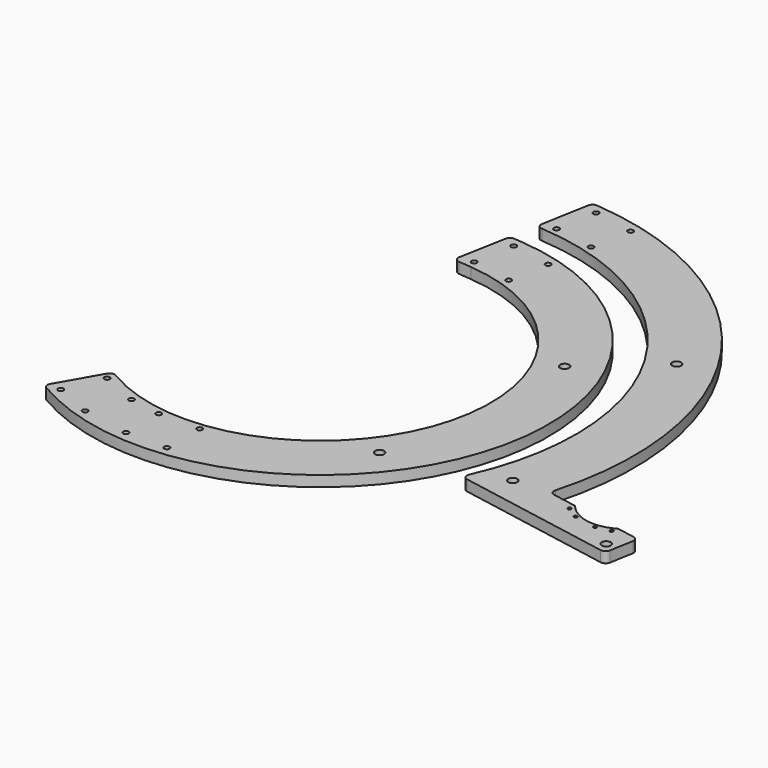
from build123d import *

# Parameters (mm, degrees)
F0_R     = 1.6
F0_R_2   = 2.65
F1_DEPTH = 6.3
F2_R     = 2.65
F2_R_2   = 1
F2_R_3   = 1.6
F3_DEPTH = 6.3


# Not quite as in the source:
# - a feature names something its author has since deleted; it is built from what else it names


with BuildPart() as f1:
    # F0 (on Top) → F1 (new body)
    with BuildSketch(Plane.XY):
        with BuildLine():
            ThreePointArc((8.7155742748, 99.6194698092), (95.3716950748, -30.0705799504), (-50, -86.6025403784))
            Line((-50, -86.6025403784), (-50.3901909826, -86.3515001966))
            Line((-50.3901909826, -86.3515001966), (-51.0879005816, -85.9026093909))
            ThreePointArc((-51.0879005816, -85.9026093909), (-53.4238831161, -85.5114532249), (-55.315580219, -86.9366899133))
            Line((-55.315580219, -86.9366899133), (-69.2410233648, -111.2966505134))
            ThreePointArc((-69.2410233648, -111.2966505134), (-69.5365488426, -113.5536105543), (-68.1625734678, -115.3683820561))
            ThreePointArc((-68.1625734678, -115.3683820561), (127.5940316963, -40.9360852487), (11.6788695282, 133.4900895443))
            Line((11.6788695282, 133.4900895443), (6.777103854, 133.918938472))
            ThreePointArc((6.777103854, 133.918938472), (4.6955895728, 133.3151874379), (3.563981512, 131.4667610231))
            Line((3.563981512, 131.4667610231), (-1.4639765495, 103.799694903))
            ThreePointArc((-1.4639765495, 103.799694903), (-0.8971544959, 101.4432412046), (1.226211336, 100.2747041633))
            Line((1.226211336, 100.2747041633), (8.7155742748, 99.6194698092))
        make_face()
        with Locations((-62.0446017151, -112.5987006942)):
            Circle(F0_R, mode=Mode.SUBTRACT)
        with Locations((-40.0351599298, -122.1686783484)):
            Circle(F0_R, mode=Mode.SUBTRACT)
        with Locations((-52.4746240608, -90.5892589089)):
            Circle(F0_R, mode=Mode.SUBTRACT)
        with Locations((-30.4651822756, -100.1592365632)):
            Circle(F0_R, mode=Mode.SUBTRACT)
        with Locations((-12, -127.3053725612)):
            Circle(F0_R, mode=Mode.SUBTRACT)
        with Locations((-12, -103.3053725612)):
            Circle(F0_R, mode=Mode.SUBTRACT)
        with Locations((12, -127.3053725612)):
            Circle(F0_R, mode=Mode.SUBTRACT)
        with Locations((12, -103.3053725612)):
            Circle(F0_R, mode=Mode.SUBTRACT)
        with Locations((91.0501851304, -70.2485856634)):
            Circle(F0_R_2, mode=Mode.SUBTRACT)
        with Locations((30.4020508273, 100.1784173637)):
            Circle(F0_R, mode=Mode.SUBTRACT)
        with Locations((6.7888099169, 104.4696705265)):
            Circle(F0_R, mode=Mode.SUBTRACT)
        with Locations((11.0800630797, 128.0829114369)):
            Circle(F0_R, mode=Mode.SUBTRACT)
        with Locations((103.8181055435, 49.4651489572)):
            Circle(F0_R_2, mode=Mode.SUBTRACT)
        with Locations((34.6933039901, 123.7916582741)):
            Circle(F0_R, mode=Mode.SUBTRACT)
    extrude(amount=F1_DEPTH)


with BuildPart() as f3:
    # F2 (on Top) → F3 (new body)
    with BuildSketch(Plane.XY):
        with BuildLine():
            ThreePointArc((7.5096449532, 153.1783445291), (8.0937160836, 150.7995084871), (10.2561765363, 149.6489587096))
            ThreePointArc((10.2561765363, 149.6489587096), (128.7199574341, 77.0141062283), (136.7163327644, -61.7142151814))
            ThreePointArc((136.7163327644, -61.7142151814), (136.7945445346, -64.3431513116), (138.9142527743, -65.9001545988))
            Line((138.9142527743, -65.9001545988), (230.5233699826, -82.5483527624))
            ThreePointArc((230.5233699826, -82.5483527624), (232.7676151982, -82.0631297717), (234.0114317417, -80.1331042939))
            Line((234.0114317417, -80.1331042939), (236.5146627534, -66.3587137629))
            ThreePointArc((236.5146627534, -66.3587137629), (236.0294397627, -64.1144685472), (234.0994142849, -62.8706520037))
            Line((234.0994142849, -62.8706520037), (223.4971377091, -60.9438917991))
            ThreePointArc((223.4971377091, -60.9438917991), (207.7144166064, -63.8990182243), (193.9805865711, -55.5798253456))
            Line((193.9805865711, -55.5798253456), (179.6486056488, -52.9752629861))
            ThreePointArc((179.6486056488, -52.9752629861), (177.6434252347, -51.6174507815), (177.2943436477, -49.2210900989))
            ThreePointArc((177.2943436477, -49.2210900989), (151.1158206101, 104.9762295062), (15.7509018567, 183.3246003424))
            ThreePointArc((15.7509018567, 183.3246003424), (13.6721883854, 182.7190260465), (12.5424385604, 180.8720189387))
            Line((12.5424385604, 180.8720189387), (7.5096449532, 153.1783445291))
        make_face()
        with Locations((155.9967381506, -53.7588847203)):
            Circle(F2_R, mode=Mode.SUBTRACT)
        with Locations((193.657645472, -59.2379068224)):
            Circle(F2_R_2, mode=Mode.SUBTRACT)
        with Locations((200.8720938117, -63.747137113)):
            Circle(F2_R_2, mode=Mode.SUBTRACT)
        with Locations((214.1726762056, -66.1642625928)):
            Circle(F2_R_2, mode=Mode.SUBTRACT)
        with Locations((228.6445281595, -76.1086358894)):
            Circle(F2_R, mode=Mode.SUBTRACT)
        with Locations((222.5123643875, -64.4816979766)):
            Circle(F2_R_2, mode=Mode.SUBTRACT)
        with Locations((39.3421615831, 149.3726692604)):
            Circle(F2_R_3, mode=Mode.SUBTRACT)
        with Locations((15.7289206727, 153.6639224232)):
            Circle(F2_R_3, mode=Mode.SUBTRACT)
        with Locations((20.0201738355, 177.2771633336)):
            Circle(F2_R_3, mode=Mode.SUBTRACT)
        with Locations((43.6334147459, 172.9859101708)):
            Circle(F2_R_3, mode=Mode.SUBTRACT)
        with Locations((142.4208181661, 83.3145278622)):
            Circle(F2_R, mode=Mode.SUBTRACT)
    extrude(amount=F3_DEPTH)


solid = Compound([f1.part, f3.part])
